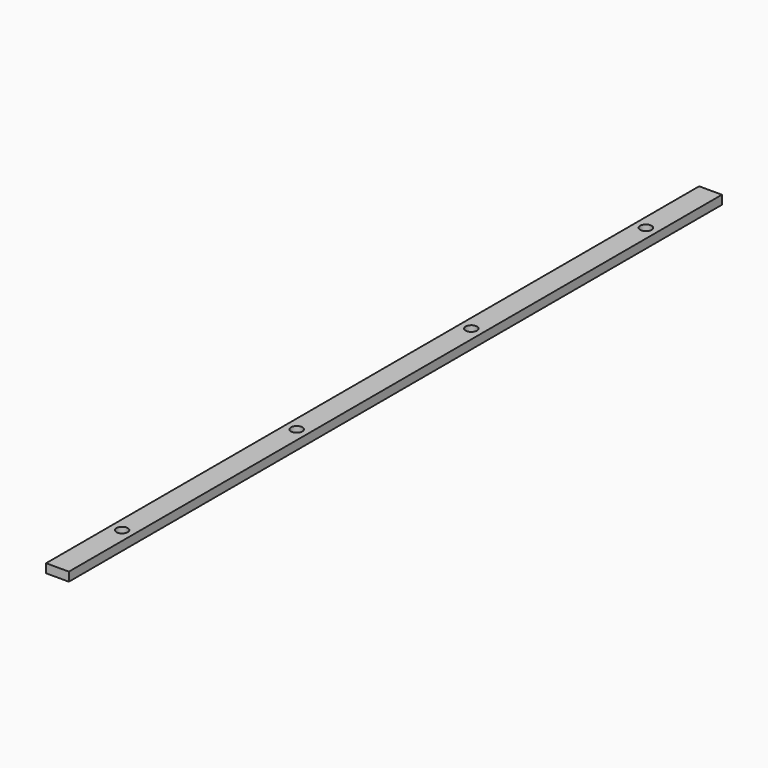
from build123d import *

# Parameters (mm, degrees)
F0_W     = 51.0843284428
F0_H     = 19.902985543
F1_DEPTH = 1828.8
F2_R     = 12.7
F3_DEPTH = 19.902985543


# Not quite as in the source:
# - a feature names something its author has since deleted; it is built from what else it names


with BuildPart() as f1:
    # F0 (on Front) → F1 (new body)
    with BuildSketch(Plane.XZ):
        with Locations((25.5421642214, 9.9514927715)):
            Rectangle(F0_W, F0_H)
    extrude(amount=F1_DEPTH)

    # F2 (on face) → F3 (cut, through all)
    with BuildSketch(Plane.XY.offset(19.902985543)):
        with Locations((25.5421642214, -1158.875)):
            Circle(F2_R)
        with Locations((25.5421642214, -669.925)):
            Circle(F2_R)
        with Locations((25.5421642214, -180.975)):
            Circle(F2_R)
        with Locations((25.5421642214, -1647.825)):
            Circle(F2_R)
    extrude(amount=-F3_DEPTH, mode=Mode.SUBTRACT)


solid = f1.part
